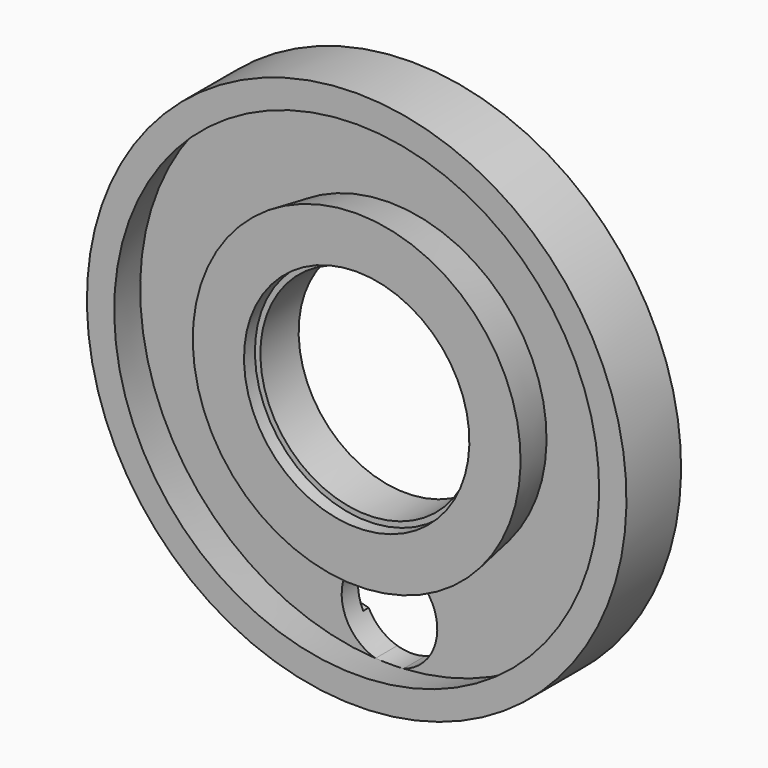
from build123d import *

# Parameters (mm, degrees)
F2_R     = 7
F3_DEPTH = 4.001


# Not quite as in the source:
# - a feature names something its author has since deleted; it is built from what else it names


with BuildPart() as f1:
    # F0 (on Right) → F1 (revolve)
    with BuildSketch(Plane.YZ):
        Polygon((-59.0552871114, 24), (-59.0552871114, 16.5), (-57.0552871114, 16.5), (-57.0552871114, 15.7), (-50.0552871114, 15.7), (-50.0552871114, 33.5), (-49.0552871114, 33.5), (-49.0552871114, 39.5), (-59.0552871114, 39.5), (-59.0552871114, 35.5), (-53.0552871114, 36.5), (-53.0552871114, 23), align=None)
    revolve(axis=Axis((0, -43.8180491328, 0), (0, 1, 0)))

    # F2 (on face) → F3 (cut, through all)
    with BuildSketch(Plane.XZ.offset(53.0552871114)):
        with Locations((0, -29.75)):
            Circle(F2_R)
        with BuildLine():
            ThreePointArc((-2.0528271341, -36.4422268908), (0, -36.75), (2.0528271341, -36.4422268908))
            ThreePointArc((2.0528271341, -36.4422268908), (0, -36.5), (-2.0528271341, -36.4422268908))
        make_face()
    extrude(amount=-F3_DEPTH, mode=Mode.SUBTRACT)


solid = f1.part
